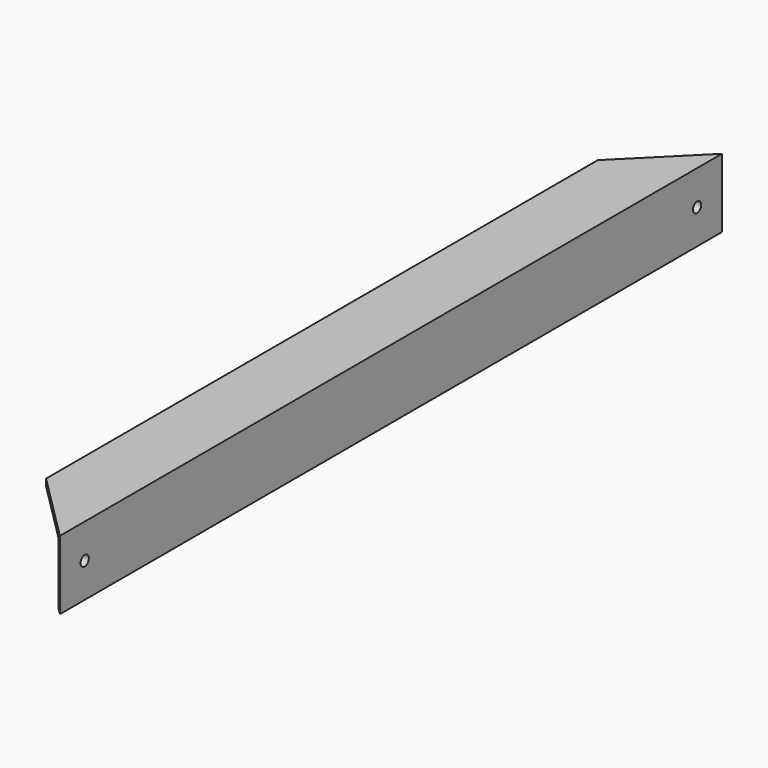
from build123d import *

# Parameters (mm, degrees)
F1_DEPTH = 120
F2_SIZE  = 19.99999
F3_R     = 1.5
F4_DEPTH = 20.001


# Not quite as in the source:
# - a fillet or chamfer is up to 0.001 mm smaller than in the source, because OpenCascade refuses the exact size


with BuildPart() as f1:
    # F0 (on Front) → F1 (new body, symmetric)
    with BuildSketch(Plane.XZ):
        Polygon((-2, 0), (0, 0), (0, 20), (-20, 20), (-20, 18), (-2, 18), align=None)
    extrude(amount=F1_DEPTH, both=True)

    # F2 (size 20 in the source; OpenCascade refuses exactly that, so slightly less here)
    f2_edges = [f1.edges().sort_by_distance(p)[0] for p in [
        (-20, -120, 19),
        (-20, 120, 19),
    ]]
    chamfer(f2_edges, length=F2_SIZE)

    # F3 (on face) → F4 (cut, through all)
    with BuildSketch(Plane.YZ):
        with Locations((111, 10)):
            Circle(F3_R)
        with Locations((-111, 10)):
            Circle(F3_R)
    extrude(amount=-F4_DEPTH, mode=Mode.SUBTRACT)


solid = f1.part
